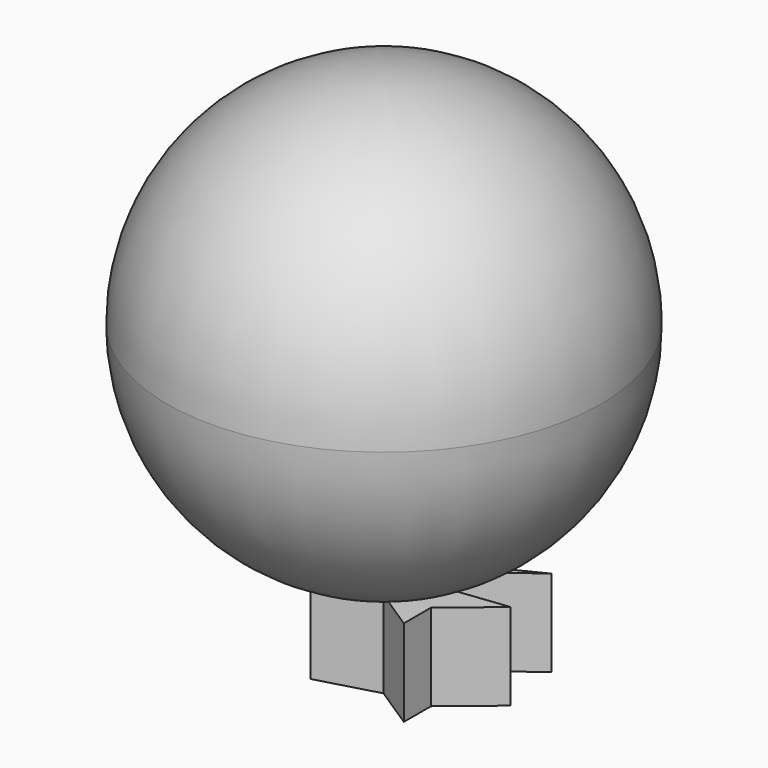
from build123d import *

# Parameters (mm, degrees)
F0_R     = 63.5
F1_DEPTH = 127
F2_R     = 63.49999
F4_DEPTH = 25.4


# Not quite as in the source:
# - a fillet or chamfer is up to 0.001 mm smaller than in the source, because OpenCascade refuses the exact size


with BuildPart() as f1:
    # F0 (on Top) → F1 (new body)
    with BuildSketch(Plane.XY):
        Circle(F0_R)
    extrude(amount=F1_DEPTH)

    # F2 (radius 63.5 in the source; OpenCascade refuses exactly that, so slightly less here)
    f2_edges = [f1.edges().sort_by_distance(p)[0] for p in [
        (-63.5, 0, 127),
        (-63.5, 0, 0),
    ]]
    fillet(f2_edges, radius=F2_R)


with BuildPart() as f4:
    # F3 (on Top) → F4 (new body)
    with BuildSketch(Plane.XY):
        Polygon((33.9144729078, 3.948839847), (0, 0), (30.8416392654, 22.6774998009), (4.1026077233, 9.2461546883), (0, 26.2496955693), (-10.0936284289, 0), (-10.0936284289, -14.3382111564), (7.42232427, -9.4631966203), (19.8794659227, -17.5901502371), (19.8794659227, -7.6642166823), align=None)
    extrude(amount=-F4_DEPTH)


solid = Compound([f1.part, f4.part])
